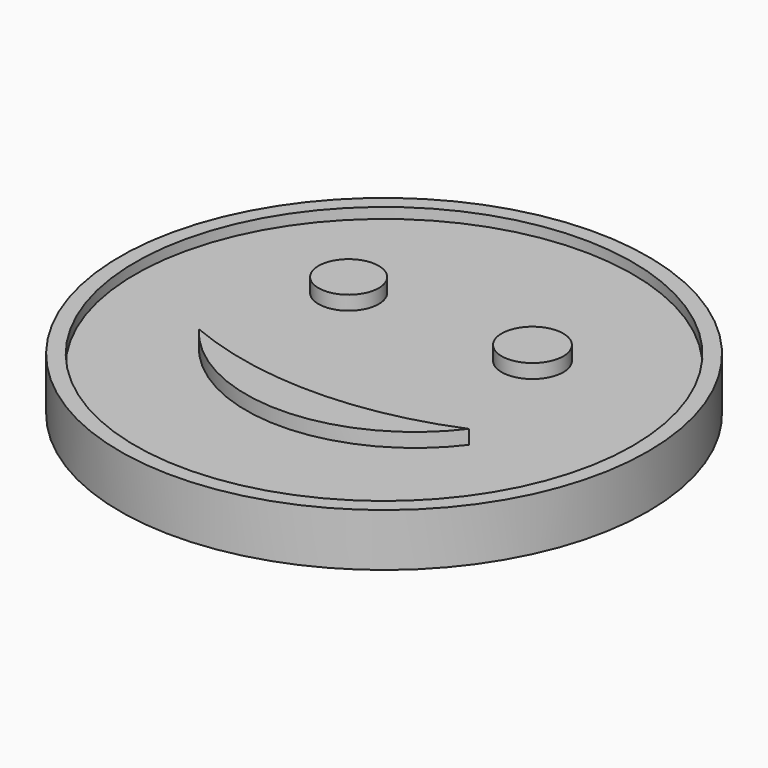
from build123d import *

# Parameters (mm, degrees)
F0_R         = 19.05
F1_DEPTH     = 3.81
F2_R         = 17.944413241
F3_DEPTH     = 0.762
F5_R         = 18.1282744633
F6_DEPTH     = 0.762
F7_TEXT_SIZE = 6.4869938392
F8_DEPTH     = 0.762
F4_R         = 2.1744064546
F4_R_2       = 2.2236914933
F9_DEPTH     = 1.016


# Not quite as in the source:
# - Text() gives the source's letters only with a copy of the font that has no kerning and outlines rounded to 1/6400 em; it was checked with that copy


with BuildPart() as f1:
    # F0 (on Top) → F1 (new body)
    with BuildSketch(Plane.XY):
        Circle(F0_R)
    extrude(amount=F1_DEPTH)

    # F2 (on face) → F3 (cut)
    with BuildSketch(Plane.XY.offset(3.81)):
        Circle(F2_R)
    extrude(amount=-F3_DEPTH, mode=Mode.SUBTRACT)

    # F5 (on face) → F6 (cut)
    with BuildSketch(Plane(origin=(0, 0, 0), x_dir=(1, 0, 0), z_dir=(0, 0, -1))):
        Circle(F5_R)
    extrude(amount=-F6_DEPTH, mode=Mode.SUBTRACT)

    # F7 (on face) → F8 (join)
    with BuildSketch(Plane(origin=(0, 0, 0.762), x_dir=(1, 0, 0), z_dir=(0, 0, -1))):
        with Locations((-16.3372771422, 0)):
            Text('People &', F7_TEXT_SIZE, font='Open Sans', text_align=(TextAlign.LEFT, TextAlign.BOTTOM))
        with Locations((-16.3372771422, -8.8223116214)):
            Text('Chocolate!', F7_TEXT_SIZE, font='Open Sans', text_align=(TextAlign.LEFT, TextAlign.BOTTOM))
    extrude(amount=F8_DEPTH)

    # F4 (on face) → F9 (join)
    with BuildSketch(Plane.XY.offset(3.048)):
        with Locations((-7.1284859441, 5.7124518789)):
            Circle(F4_R)
        with Locations((6.1403526925, 5.7124518789)):
            Circle(F4_R_2)
        with BuildLine():
            ThreePointArc((9.7485454753, -4.5301602222), (0, -6.4889750752), (-9.7485454753, -4.5301602222))
            ThreePointArc((-9.7485454753, -4.5301602222), (0, -9.3958968888), (9.7485454753, -4.5301602222))
        make_face()
    extrude(amount=F9_DEPTH)


solid = f1.part
